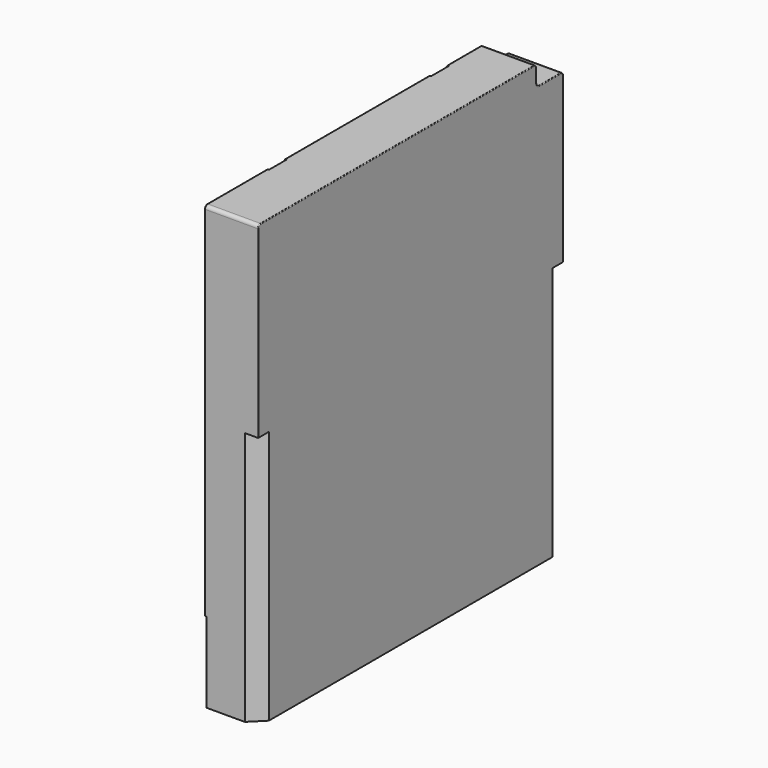
from build123d import *

# Parameters (mm, degrees)
F1_DEPTH  = 3.875
F3_DEPTH  = 38
F4_W      = 27
F4_H      = 54
F4_W_2    = 20
F4_H_2    = 4
F4_W_3    = 11.7
F5_DEPTH  = 0.25
F8_R      = 0.5
F9_R      = 0.1
F11_W     = 7.15
F11_H     = 50
F12_DEPTH = 62
F14_DEPTH = 3


# Not quite as in the source:
# - a pattern or mirror of a feature is missing from the dataset's text; its kind, count and spacing are read off the source's solid


with BuildPart() as f1:
    # F0 (on Right) → F1 (new body, symmetric)
    with BuildSketch(Plane.YZ):
        Polygon((23.5, 33), (-28.5, 33), (-28.5, -33), (28.5, -33), (28.5, 30), (23.5, 30), align=None)
    extrude(amount=F1_DEPTH, both=True)

    # F2 (on face) → F3 (cut)
    with BuildSketch(Plane(origin=(0, 0, -33), x_dir=(1, 0, 0), z_dir=(0, 0, -1))):
        Polygon((3.875, 28.5), (1.875, 28.5), (3.875, 26.5), align=None)
        Polygon((3.875, -26.5), (1.875, -28.5), (3.875, -28.5), align=None)
    extrude(amount=-F3_DEPTH, mode=Mode.SUBTRACT)

    # F4 (on face) → F5 (join)
    with BuildSketch(Plane(origin=(-3.875, 0, 0), x_dir=(0, -1, 0), z_dir=(-1, 0, 0))):
        with Locations((0, 6)):
            Rectangle(F4_W, F4_H)
        with Locations((0, 29)):
            Rectangle(F4_W_2, F4_H_2, mode=Mode.SUBTRACT)
        with Locations((22.65, 6)):
            Rectangle(F4_W_3, F4_H)
        Polygon((-28.5, 30), (-28.5, -21), (-16.8, -21), (-16.8, 33), (-23.5, 33), (-23.5, 30), align=None)
    extrude(amount=F5_DEPTH)

    # F8
    f8_edges = [f1.edges().sort_by_distance(p)[0] for p in [
        (-0.125, 23.5, 33),
        (-0.125, 23.5, 30),
        (-0.125, 28.5, 30),
        (-0.125, -28.5, 33),
    ]]
    fillet(f8_edges, radius=F8_R)

    # F9
    f9_edges = [f1.edges().sort_by_distance(p)[0] for p in [
        (3.875, -2.5, 33),
        (3.875, 26, 30),
        (-4.125, 26, 30),
        (-4.125, 23.5, 31.5),
        (3.875, 23.5, 31.5),
        (-4.125, 19.9, 33),
        (-4.125, 0, 33),
        (-4.125, -22.4, 33),
        (-4.125, -28.5, 5.75),
        (3.875, -28.5, 18.75),
        (-4.125, 28.5, 4.25),
        (-4.125, -28.353553, 32.853553),
        (3.875, -28.353553, 32.853553),
        (3.875, 23.646447, 30.146447),
        (3.875, 23.353553, 32.853553),
        (3.875, 28.353553, 29.853553),
        (3.875, 28.5, 17.25),
        (-4.125, 23.353553, 32.853553),
        (-4.125, 28.353553, 29.853553),
        (-4.125, 23.646447, 30.146447),
    ]]
    fillet(f9_edges, radius=F9_R)

    # F11 (on face) → F12 (cut)
    with BuildSketch(Plane(origin=(0, 0, -33), x_dir=(1, 0, 0), z_dir=(0, 0, -1))):
        Rectangle(F11_W, F11_H)
    extrude(amount=-F12_DEPTH, mode=Mode.SUBTRACT)

    # F13 (on face) → F14 (cut)
    with BuildSketch(Plane(origin=(0, 0, -33), x_dir=(1, 0, 0), z_dir=(0, 0, -1))):
        with BuildLine():
            Line((3.575, -25), (-3.575, -25))
            Line((-3.575, -25), (-3.575, -26))
            ThreePointArc((-3.575, -26), (-3.5017766953, -26.1767766953), (-3.325, -26.25))
            Line((-3.325, -26.25), (3.325, -26.25))
            ThreePointArc((3.325, -26.25), (3.5017766953, -26.1767766953), (3.575, -26))
            Line((3.575, -26), (3.575, -25))
        make_face()
    f14 = extrude(amount=-F14_DEPTH, mode=Mode.SUBTRACT)

    # F14_copies: F14 across plane
    add(f14.mirror(Plane(origin=(0, 0, 0), x_dir=(0, 0, -1), z_dir=(0, -1, 0))), mode=Mode.SUBTRACT)


solid = f1.part
